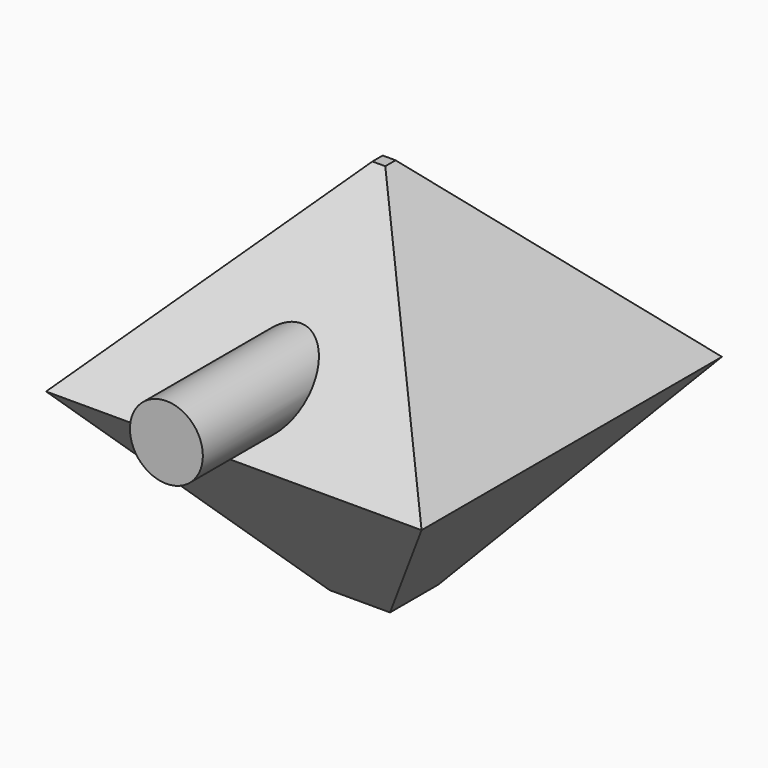
from build123d import *

# Parameters (mm, degrees)
F0_W          = 25.4
F0_H          = 25.4
F1_DEPTH      = 12.7
F1_TAPER      = 44
F1_DEPTH_BACK = 12.7
F1_TAPER_BACK = 40
F4_R          = 2.4668043614
F5_DEPTH      = 14.478


with BuildPart() as f1:
    # F0 (on Top) → F1 (new body, two sides)
    with BuildSketch(Plane.XY) as f1_sk:
        Rectangle(F0_W, F0_H)
    extrude(amount=F1_DEPTH, taper=F1_TAPER)
    extrude(f1_sk.sketch, amount=-F1_DEPTH_BACK, taper=F1_TAPER_BACK)

    # F4 (on face) → F5 (join)
    with BuildSketch(Plane.XZ.offset(3.9232242852)):
        with Locations((0, 3.4155005123)):
            Circle(F4_R)
    extrude(amount=F5_DEPTH)


solid = f1.part
